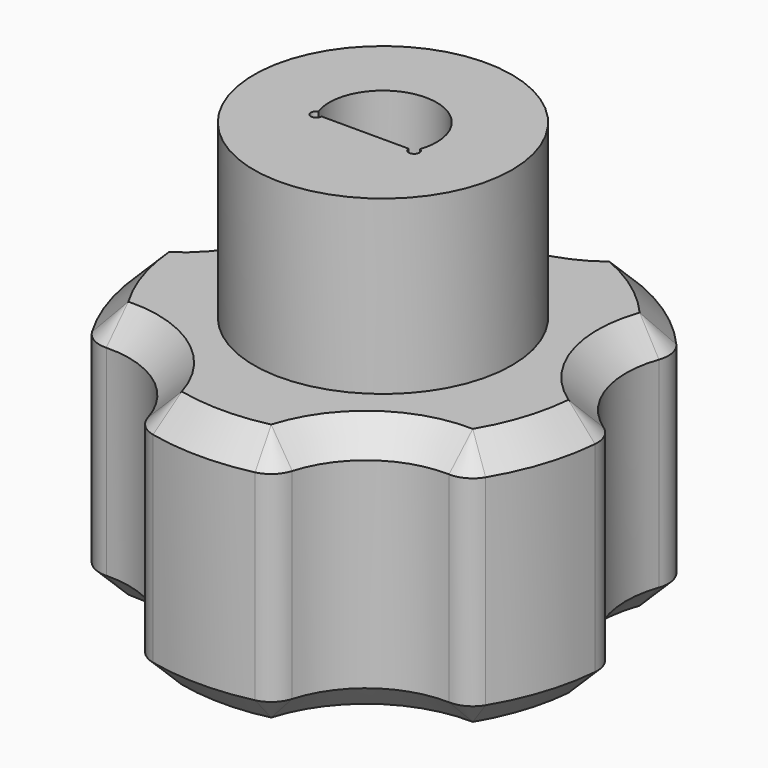
from build123d import *

# Parameters (mm, degrees)
F1_R      = 9
F2_DEPTH  = 12
F2_FACE_R = 9
F3_DEPTH  = 18
F5_DEPTH  = 12
F6_SIZE   = 1.99999


# Not quite as in the source:
# - a fillet or chamfer is up to 0.001 mm smaller than in the source, because OpenCascade refuses the exact size


with BuildPart() as f2:
    # F1 (on Top) → F2 (new body)
    with BuildSketch(Plane.XY):
        Circle(F1_R)
        with BuildLine():
            ThreePointArc((-3.5524069735, -1.2012096798), (-0.6086763711, 3.7002720272), (3.75, 0))
            ThreePointArc((3.75, 0), (3.7002720272, -0.6086763711), (3.5524069735, -1.2012096798))
            ThreePointArc((3.5524069735, -1.2012096798), (3.7247345197, -1.339079143), (3.7896742158, -1.55))
            ThreePointArc((3.7896742158, -1.55), (3.6098282416, -1.8702185288), (3.242794716, -1.8832903202))
            ThreePointArc((3.242794716, -1.8832903202), (0, -3.75), (-3.242794716, -1.8832903202))
            ThreePointArc((-3.242794716, -1.8832903202), (-3.7561416374, -1.705), (-3.5524069735, -1.2012096798))
        make_face(mode=Mode.SUBTRACT)
        with BuildLine():
            Line((3.0396742158, -1.55), (-3.0396742158, -1.55))
            ThreePointArc((-3.0396742158, -1.55), (-3.0944556869, -1.7451540258), (-3.242794716, -1.8832903202))
            ThreePointArc((-3.242794716, -1.8832903202), (0, -3.75), (3.242794716, -1.8832903202))
            ThreePointArc((3.242794716, -1.8832903202), (3.0944556869, -1.7451540258), (3.0396742158, -1.55))
        make_face()
    extrude(amount=F2_DEPTH)

    # F1 (on Top) + F2_face (on face) → F3 (join)
    with BuildSketch(Plane.XY):
        with BuildLine():
            ThreePointArc((-4.2766728371, 14.4583333333), (-5.2456206791, 14.8589384831), (-6.2840906994, 14.7142857143))
            ThreePointArc((-6.2840906994, 14.7142857143), (-9.4045640367, 12.94427191), (-12.0522264909, 10.5234897545))
            ThreePointArc((-12.0522264909, 10.5234897545), (-12.5107043337, 9.5805462385), (-12.4291275454, 8.5352282801))
            ThreePointArc((-12.4291275454, 8.5352282801), (-12.3637347118, 4.0172209269), (-15.0722567175, 0.4005131406))
            ThreePointArc((-15.0722567175, 0.4005131406), (-15.7526762055, -0.3972172192), (-15.9360081315, -1.4295610629))
            ThreePointArc((-15.9360081315, -1.4295610629), (-15.2169042607, -4.94427191), (-13.7327763109, -8.2104113658))
            ThreePointArc((-13.7327763109, -8.2104113658), (-12.9776611805, -8.9378352769), (-11.9582961107, -9.1832721545))
            ThreePointArc((-11.9582961107, -9.1832721545), (-7.6412082798, -10.5172209269), (-5.0384941015, -14.2108025995))
            ThreePointArc((-5.0384941015, -14.2108025995), (-4.4900686296, -15.1044322255), (-3.5649039709, -15.5978030401))
            ThreePointArc((-3.5649039709, -15.5978030401), (0, -16), (3.5649039709, -15.5978030401))
            ThreePointArc((3.5649039709, -15.5978030401), (4.4900686296, -15.1044322255), (5.0384941015, -14.2108025995))
            ThreePointArc((5.0384941015, -14.2108025995), (7.6412082798, -10.5172209269), (11.9582961107, -9.1832721545))
            ThreePointArc((11.9582961107, -9.1832721545), (12.9776611805, -8.9378352769), (13.7327763109, -8.2104113658))
            ThreePointArc((13.7327763109, -8.2104113658), (15.2169042607, -4.94427191), (15.9360081315, -1.4295610629))
            ThreePointArc((15.9360081315, -1.4295610629), (15.7526762055, -0.3972172192), (15.0722567175, 0.4005131406))
            ThreePointArc((15.0722567175, 0.4005131406), (12.3637347118, 4.0172209269), (12.4291275454, 8.5352282801))
            ThreePointArc((12.4291275454, 8.5352282801), (12.5107043337, 9.5805462385), (12.0522264909, 10.5234897545))
            ThreePointArc((12.0522264909, 10.5234897545), (9.4045640367, 12.94427191), (6.2840906994, 14.7142857143))
            ThreePointArc((6.2840906994, 14.7142857143), (5.2456206791, 14.8589384831), (4.2766728371, 14.4583333333))
            ThreePointArc((4.2766728371, 14.4583333333), (0, 13), (-4.2766728371, 14.4583333333))
        make_face()
        Circle(F1_R, mode=Mode.SUBTRACT)
        with BuildLine():
            ThreePointArc((3.5524069735, -1.2012096798), (3.7002720272, -0.6086763711), (3.75, 0))
            ThreePointArc((3.75, 0), (-0.6086763711, 3.7002720272), (-3.5524069735, -1.2012096798))
            ThreePointArc((-3.5524069735, -1.2012096798), (-3.2037533587, -1.2399396961), (-3.0396742158, -1.55))
            Line((-3.0396742158, -1.55), (3.0396742158, -1.55))
            ThreePointArc((3.0396742158, -1.55), (3.2037533587, -1.2399396961), (3.5524069735, -1.2012096798))
        make_face()
        with BuildLine():
            ThreePointArc((-3.4146742158, -1.55), (-3.487903202, -1.3773275768), (-3.5524069735, -1.2012096798))
            ThreePointArc((-3.5524069735, -1.2012096798), (-3.7561416374, -1.705), (-3.242794716, -1.8832903202))
            ThreePointArc((-3.242794716, -1.8832903202), (-3.332903202, -1.7187949983), (-3.4146742158, -1.55))
        make_face()
        with BuildLine():
            ThreePointArc((-3.0396742158, -1.55), (-3.2037533587, -1.2399396961), (-3.5524069735, -1.2012096798))
            ThreePointArc((-3.5524069735, -1.2012096798), (-3.487903202, -1.3773275768), (-3.4146742158, -1.55))
            Line((-3.4146742158, -1.55), (-3.0396742158, -1.55))
        make_face()
        with BuildLine():
            Line((-3.0396742158, -1.55), (-3.4146742158, -1.55))
            ThreePointArc((-3.4146742158, -1.55), (-3.332903202, -1.7187949983), (-3.242794716, -1.8832903202))
            ThreePointArc((-3.242794716, -1.8832903202), (-3.0944556869, -1.7451540258), (-3.0396742158, -1.55))
        make_face()
        with BuildLine():
            ThreePointArc((3.4146742158, -1.55), (3.487903202, -1.3773275768), (3.5524069735, -1.2012096798))
            ThreePointArc((3.5524069735, -1.2012096798), (3.2037533587, -1.2399396961), (3.0396742158, -1.55))
            Line((3.0396742158, -1.55), (3.4146742158, -1.55))
        make_face()
        with BuildLine():
            ThreePointArc((3.242794716, -1.8832903202), (3.332903202, -1.7187949983), (3.4146742158, -1.55))
            Line((3.4146742158, -1.55), (3.0396742158, -1.55))
            ThreePointArc((3.0396742158, -1.55), (3.0944556869, -1.7451540258), (3.242794716, -1.8832903202))
        make_face()
        with BuildLine():
            ThreePointArc((3.7896742158, -1.55), (3.7247345197, -1.339079143), (3.5524069735, -1.2012096798))
            ThreePointArc((3.5524069735, -1.2012096798), (3.487903202, -1.3773275768), (3.4146742158, -1.55))
            ThreePointArc((3.4146742158, -1.55), (3.332903202, -1.7187949983), (3.242794716, -1.8832903202))
            ThreePointArc((3.242794716, -1.8832903202), (3.6098282416, -1.8702185288), (3.7896742158, -1.55))
        make_face()
    with BuildSketch(Plane(origin=(0, -0.1158950357, 12), x_dir=(1, 0, 0), z_dir=(0, 0, 1))):
        with Locations((0, 0.1158950357)):
            Circle(F2_FACE_R)
        with BuildLine():
            ThreePointArc((-3.5524069735, -1.0853146441), (0, 3.8658950357), (3.5524069735, -1.0853146441))
            ThreePointArc((3.5524069735, -1.0853146441), (3.6255950728, -1.7441652682), (3.0396742158, -1.4341049643))
            Line((3.0396742158, -1.4341049643), (-3.0396742158, -1.4341049643))
            ThreePointArc((-3.0396742158, -1.4341049643), (-3.6255950728, -1.7441652682), (-3.5524069735, -1.0853146441))
        make_face(mode=Mode.SUBTRACT)
    extrude(amount=F3_DEPTH)

    # F4 (on face) → F5 (cut)
    with BuildSketch(Plane.XY.offset(18)):
        with BuildLine():
            ThreePointArc((2.891366459, -0.8), (2.9727175595, -0.4036710437), (3, 0))
            ThreePointArc((3, 0), (-0.4036710437, 2.9727175595), (-2.891366459, -0.8))
            Line((-2.891366459, -0.8), (2.891366459, -0.8))
        make_face()
    extrude(amount=-F5_DEPTH, mode=Mode.SUBTRACT)

    # F6 (size 2 in the source; OpenCascade refuses exactly that, so slightly less here)
    f6_edges = [f2.edges().sort_by_distance(p)[0] for p in [
        (0, -16, 18),
        (0, -16, 0),
    ]]
    chamfer(f6_edges, length=F6_SIZE)


solid = f2.part
